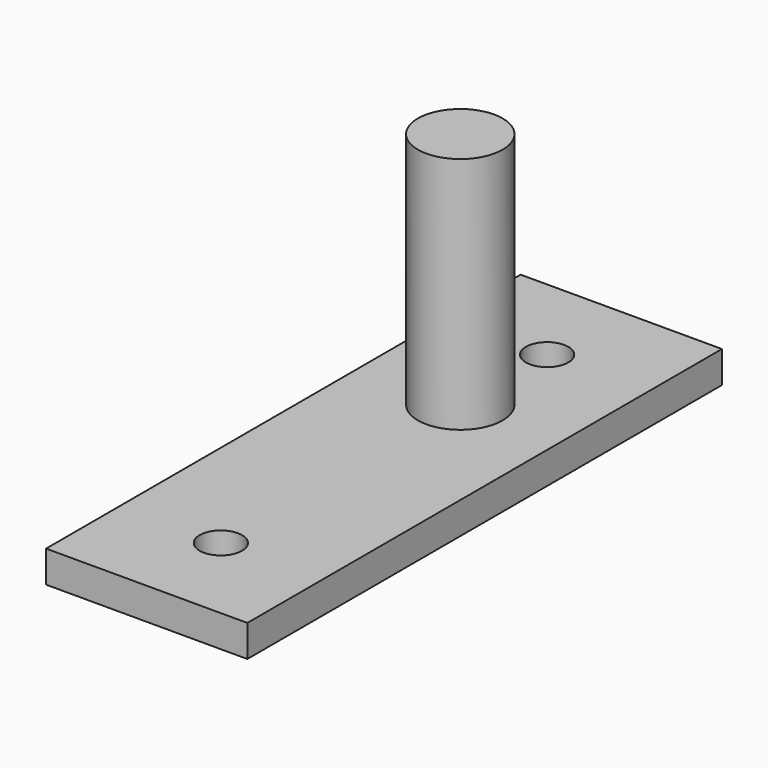
from build123d import *

# Parameters (mm, degrees)
F1_DEPTH = 6
F2_R     = 4
F3_DEPTH = 6.001
F4_R     = 8
F5_DEPTH = 45


# Not quite as in the source:
# - a feature names something its author has since deleted; it is built from what else it names


with BuildPart() as f1:
    # F0 (on Top) → F1 (new body)
    with BuildSketch(Plane.XY):
        Polygon((-19, 56), (-19, 0), (-19, -56), (0, -56), (19, -56), (19, 0), (19, 56), (0, 56), align=None)
    extrude(amount=F1_DEPTH)

    # F2 (on face) → F3 (cut, through all)
    with BuildSketch(Plane.XY.offset(6)):
        with Locations((0, 38.5)):
            Circle(F2_R)
        with Locations((0, -38.5)):
            Circle(F2_R)
    extrude(amount=-F3_DEPTH, mode=Mode.SUBTRACT)

    # F4 (on face) → F5 (join)
    with BuildSketch(Plane.XY.offset(6)):
        with Locations((0, 18)):
            Circle(F4_R)
    extrude(amount=F5_DEPTH)


solid = f1.part
